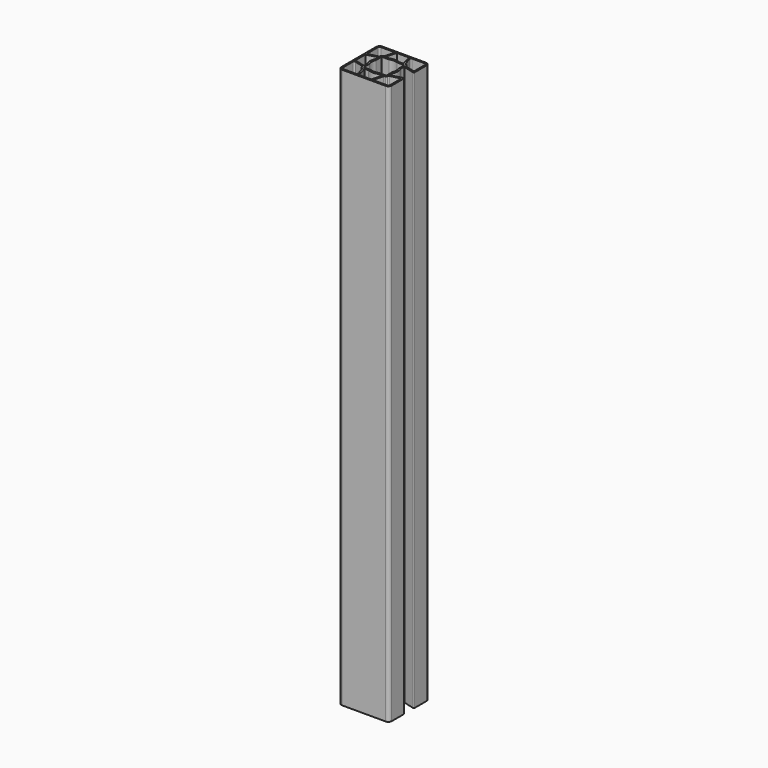
from build123d import *

# Parameters (mm, degrees)
F1_DEPTH = 1000


# Not quite as in the source:
# - ends of sketch curves that miss each other by under 0.0002 mm in the source are joined


with BuildPart() as f1:
    # F0 (on Top) → F1 (new body)
    with BuildSketch(Plane.XY):
        with BuildLine():
            Line((23, 9.273618), (23, 14.841657))
            ThreePointArc((23, 14.841657), (23.3912385359, 15.6350103133), (24.2588189596, 15.8075828492))
            Line((24.2588189596, 15.8075828492), (43.426476, 10.671624))
            ThreePointArc((43.426476, 10.671624), (44.5109517857, 10.8873403242), (45, 11.879032))
            Line((45, 11.879032), (45, 39))
            ThreePointArc((45, 39), (43.2426406871, 43.2426406871), (39, 45))
            Line((39, 45), (-39, 45))
            ThreePointArc((-39, 45), (-43.2426406871, 43.2426406871), (-45, 39))
            Line((-45, 39), (-45, -39))
            ThreePointArc((-45, -39), (-43.2426406871, -43.2426406871), (-39, -45))
            Line((-39, -45), (39, -45))
            ThreePointArc((39, -45), (43.2426406871, -43.2426406871), (45, -39))
            Line((45, -39), (45, -11.879032))
            ThreePointArc((45, -11.879032), (44.5109517857, -10.8873403242), (43.4264761923, -10.6716247175))
            Line((43.4264761923, -10.6716247175), (24.258819, -15.807583))
            ThreePointArc((24.258819, -15.807583), (23.3912385359, -15.6350103133), (23, -14.841657))
            Line((23, -14.841657), (23, -9.273618))
            ThreePointArc((23, -9.273618), (23.022474706, -9.062799833), (23.0888885991, -8.8614578186))
            ThreePointArc((23.0888885991, -8.8614578186), (25, 0), (23.0888887851, 8.8614579028))
            ThreePointArc((23.0888887851, 8.8614579028), (23.022474706, 9.062799833), (23, 9.273618))
        make_face()
        with BuildLine():
            Line((15.807583, -24.258819), (10.98686, -42.25))
            Line((10.98686, -42.25), (-10.98686, -42.25))
            Line((-10.98686, -42.25), (-15.807583, -24.258819))
            ThreePointArc((-15.807583, -24.258819), (-15.6350103133, -23.3912385359), (-14.841657, -23))
            Line((-14.841657, -23), (-9.273618, -23))
            ThreePointArc((-9.273618, -23), (-9.062799833, -23.022474706), (-8.8614578186, -23.0888885991))
            ThreePointArc((-8.8614578186, -23.0888885991), (0, -25), (8.8614579028, -23.0888887851))
            ThreePointArc((8.8614579028, -23.0888887851), (9.062799833, -23.022474706), (9.273618, -23))
            Line((9.273618, -23), (14.841657, -23))
            ThreePointArc((14.841657, -23), (15.6350103133, -23.3912385359), (15.807583, -24.258819))
        make_face(mode=Mode.SUBTRACT)
        with BuildLine():
            ThreePointArc((-42.25, -16.440321), (-41.4675229282, -14.8536143733), (-39.7323620808, -14.5084693016))
            Line((-39.7323620808, -14.5084693016), (-24.482362, -18.594694))
            ThreePointArc((-24.482362, -18.594694), (-23.4132933733, -19.3090230718), (-23, -20.526546))
            Line((-23, -20.526546), (-23, -21))
            ThreePointArc((-23, -21), (-22.4142135624, -22.4142135624), (-21, -23))
            Line((-21, -23), (-20.526546, -23))
            ThreePointArc((-20.526546, -23), (-19.3090230718, -23.4132933733), (-18.5946943016, -24.4823620808))
            Line((-18.5946943016, -24.4823620808), (-14.508469, -39.732362))
            ThreePointArc((-14.508469, -39.732362), (-14.8536143733, -41.4675229282), (-16.440321, -42.25))
            Line((-16.440321, -42.25), (-39, -42.25))
            ThreePointArc((-39, -42.25), (-41.2980970389, -41.2980970389), (-42.25, -39))
            Line((-42.25, -39), (-42.25, -16.440321))
        make_face(mode=Mode.SUBTRACT)
        with BuildLine():
            ThreePointArc((16.440321, -42.25), (14.8536143733, -41.4675229282), (14.5084693016, -39.7323620808))
            Line((14.5084693016, -39.7323620808), (18.594694, -24.482362))
            ThreePointArc((18.594694, -24.482362), (19.3090230718, -23.4132933733), (20.526546, -23))
            Line((20.526546, -23), (21, -23))
            ThreePointArc((21, -23), (22.4142135624, -22.4142135624), (23, -21))
            Line((23, -21), (23, -20.526546))
            ThreePointArc((23, -20.526546), (23.4132933733, -19.3090230718), (24.4823620808, -18.5946943016))
            Line((24.4823620808, -18.5946943016), (39.732362, -14.508469))
            ThreePointArc((39.732362, -14.508469), (41.4675229282, -14.8536143733), (42.25, -16.440321))
            Line((42.25, -16.440321), (42.25, -39))
            ThreePointArc((42.25, -39), (41.2980970389, -41.2980970389), (39, -42.25))
            Line((39, -42.25), (16.440321, -42.25))
        make_face(mode=Mode.SUBTRACT)
        with BuildLine():
            Line((-24.258819, -15.807583), (-42.25, -10.98686))
            Line((-42.25, -10.98686), (-42.25, 10.98686))
            Line((-42.25, 10.98686), (-24.258819, 15.807583))
            ThreePointArc((-24.258819, 15.807583), (-23.3912385359, 15.6350103133), (-23, 14.841657))
            Line((-23, 14.841657), (-23, 9.273618))
            ThreePointArc((-23, 9.273618), (-23.022474706, 9.062799833), (-23.0888885991, 8.8614578186))
            ThreePointArc((-23.0888885991, 8.8614578186), (-25, 0), (-23.0888887851, -8.8614579028))
            ThreePointArc((-23.0888887851, -8.8614579028), (-23.022474706, -9.062799833), (-23, -9.273618))
            Line((-23, -9.273618), (-23, -14.841657))
            ThreePointArc((-23, -14.841657), (-23.3912385359, -15.6350103133), (-24.258819, -15.807583))
        make_face(mode=Mode.SUBTRACT)
        with BuildLine():
            ThreePointArc((19.25, 20.25), (19.9571067812, 19.9571067812), (20.25, 19.25))
            Line((20.25, 19.25), (20.25, 7.3951))
            ThreePointArc((20.25, 7.3951), (20.2639867072, 7.2284333074), (20.3055555728, 7.0664288513))
            ThreePointArc((20.3055554887, 7.066428822), (21.5, 0), (20.3055554887, -7.066428822))
            ThreePointArc((20.3055555728, -7.0664288513), (20.2639867072, -7.2284333074), (20.25, -7.3951))
            Line((20.25, -7.3951), (20.25, -19.25))
            ThreePointArc((20.25, -19.25), (19.9571067812, -19.9571067812), (19.25, -20.25))
            Line((19.25, -20.25), (7.3951, -20.25))
            ThreePointArc((7.3951, -20.25), (7.2284333074, -20.2639867072), (7.0664288513, -20.3055555728))
            ThreePointArc((7.066428822, -20.3055554887), (0, -21.5), (-7.066428822, -20.3055554887))
            ThreePointArc((-7.0664288513, -20.3055555728), (-7.2284333074, -20.2639867072), (-7.3951, -20.25))
            Line((-7.3951, -20.25), (-19.25, -20.25))
            ThreePointArc((-19.25, -20.25), (-19.9571067812, -19.9571067812), (-20.25, -19.25))
            Line((-20.25, -19.25), (-20.25, -7.3951))
            ThreePointArc((-20.25, -7.3951), (-20.2639867072, -7.2284333074), (-20.3055555728, -7.0664288513))
            ThreePointArc((-20.3055554887, -7.066428822), (-21.5, 0), (-20.3055554887, 7.066428822))
            ThreePointArc((-20.3055555728, 7.0664288513), (-20.2639867072, 7.2284333074), (-20.25, 7.3951))
            Line((-20.25, 7.3951), (-20.25, 19.25))
            ThreePointArc((-20.25, 19.25), (-19.9571067812, 19.9571067812), (-19.25, 20.25))
            Line((-19.25, 20.25), (-7.3951, 20.25))
            ThreePointArc((-7.3951, 20.25), (-7.2284333074, 20.2639867072), (-7.0664288513, 20.3055555728))
            ThreePointArc((-7.066428822, 20.3055554887), (0, 21.5), (7.066428822, 20.3055554887))
            ThreePointArc((7.0664288513, 20.3055555728), (7.2284333074, 20.2639867072), (7.3951, 20.25))
            Line((7.3951, 20.25), (19.25, 20.25))
        make_face(mode=Mode.SUBTRACT)
        with BuildLine():
            ThreePointArc((-16.440321, 42.25), (-14.8536143733, 41.4675229282), (-14.5084693016, 39.7323620808))
            Line((-14.5084693016, 39.7323620808), (-18.594694, 24.482362))
            ThreePointArc((-18.594694, 24.482362), (-19.3090230718, 23.4132933733), (-20.526546, 23))
            Line((-20.526546, 23), (-21, 23))
            ThreePointArc((-21, 23), (-22.4142135624, 22.4142135624), (-23, 21))
            Line((-23, 21), (-23, 20.526546))
            ThreePointArc((-23, 20.526546), (-23.4132933733, 19.3090230718), (-24.4823620808, 18.5946943016))
            Line((-24.4823620808, 18.5946943016), (-39.732362, 14.508469))
            ThreePointArc((-39.732362, 14.508469), (-41.4675229282, 14.8536143733), (-42.25, 16.440321))
            Line((-42.25, 16.440321), (-42.25, 39))
            ThreePointArc((-42.25, 39), (-41.2980970389, 41.2980970389), (-39, 42.25))
            Line((-39, 42.25), (-16.440321, 42.25))
        make_face(mode=Mode.SUBTRACT)
        with BuildLine():
            ThreePointArc((15.8075828492, 24.2588189596), (15.6350103133, 23.3912385359), (14.841657, 23))
            Line((14.841657, 23), (9.273618, 23))
            ThreePointArc((9.273618, 23), (9.062799833, 23.022474706), (8.8614578186, 23.0888885991))
            ThreePointArc((8.8614578186, 23.0888885991), (0, 25), (-8.8614579028, 23.0888887851))
            ThreePointArc((-8.8614579028, 23.0888887851), (-9.062799833, 23.022474706), (-9.273618, 23))
            Line((-9.273618, 23), (-14.841657, 23))
            ThreePointArc((-14.841657, 23), (-15.6350103133, 23.3912385359), (-15.8075828492, 24.2588189596))
            Line((-15.8075828492, 24.2588189596), (-10.98686, 42.25))
            Line((-10.98686, 42.25), (10.98686, 42.25))
            Line((10.98686, 42.25), (15.8075828492, 24.2588189596))
        make_face(mode=Mode.SUBTRACT)
        with BuildLine():
            ThreePointArc((42.25, 16.440321), (41.4675229282, 14.8536143733), (39.7323620808, 14.5084693016))
            Line((39.7323620808, 14.5084693016), (24.482362, 18.594694))
            ThreePointArc((24.482362, 18.594694), (23.4132933733, 19.3090230718), (23, 20.526546))
            Line((23, 20.526546), (23, 21))
            ThreePointArc((23, 21), (22.4142135624, 22.4142135624), (21, 23))
            Line((21, 23), (20.526546, 23))
            ThreePointArc((20.526546, 23), (19.3090230718, 23.4132933733), (18.5946943016, 24.4823620808))
            Line((18.5946943016, 24.4823620808), (14.508469, 39.732362))
            ThreePointArc((14.508469, 39.732362), (14.8536143733, 41.4675229282), (16.440321, 42.25))
            Line((16.440321, 42.25), (39, 42.25))
            ThreePointArc((39, 42.25), (41.2980970389, 41.2980970389), (42.25, 39))
            Line((42.25, 39), (42.25, 16.440321))
        make_face(mode=Mode.SUBTRACT)
    extrude(amount=F1_DEPTH)


solid = f1.part
